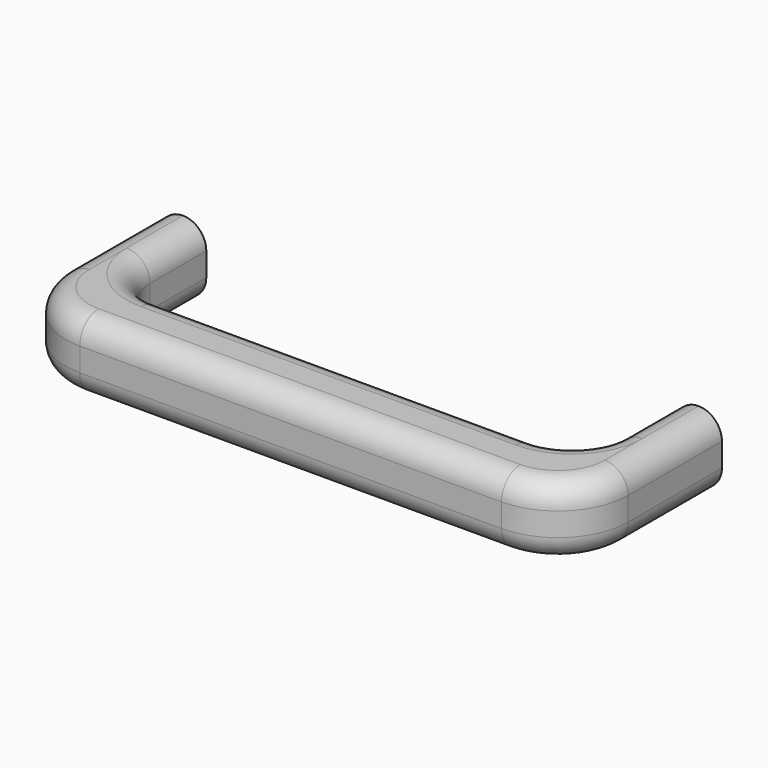
from build123d import *

# Parameters (mm, degrees)
F1_DEPTH = 7.5
F2_R     = 4.99999


# Not quite as in the source:
# - a fillet or chamfer is up to 0.001 mm smaller than in the source, because OpenCascade refuses the exact size


with BuildPart() as f1:
    # F0 (on Top) → F1 (new body, symmetric)
    with BuildSketch(Plane.XY):
        with BuildLine():
            ThreePointArc((-68.4076752503, 15.1665699541), (-64.0142769681, 4.5599682363), (-53.4076752503, 0.1665699541))
            Line((-53.4076752503, 0.1665699541), (36.5923247497, 0.1665699541))
            ThreePointArc((36.5923247497, 0.1665699541), (47.1989264675, 4.5599682363), (51.5923247497, 15.1665699541))
            Line((51.5923247497, 15.1665699541), (51.5923247497, 40.1665699541))
            Line((51.5923247497, 40.1665699541), (41.5923247497, 40.1665699541))
            Line((41.5923247497, 40.1665699541), (41.5923247497, 25.1665699541))
            ThreePointArc((41.5923247497, 25.1665699541), (38.6633925615, 18.0955021423), (31.5923247497, 15.1665699541))
            Line((31.5923247497, 15.1665699541), (-48.4076752503, 15.1665699541))
            ThreePointArc((-48.4076752503, 15.1665699541), (-55.4787430622, 18.0955021423), (-58.4076752503, 25.1665699541))
            Line((-58.4076752503, 25.1665699541), (-58.4076752503, 40.1665699541))
            Line((-58.4076752503, 40.1665699541), (-68.4076752503, 40.1665699541))
            Line((-68.4076752503, 40.1665699541), (-68.4076752503, 15.1665699541))
        make_face()
    extrude(amount=F1_DEPTH, both=True)

    # F2 (radius 5 in the source; OpenCascade refuses exactly that, so slightly less here)
    f2_edges = [f1.edges().sort_by_distance(p)[0] for p in [
        (-8.407675, 15.16657, 7.5),
        (-8.407675, 0.16657, 7.5),
        (-8.407675, 0.16657, -7.5),
        (-8.407675, 15.16657, -7.5),
    ]]
    fillet(f2_edges, radius=F2_R)


solid = f1.part
